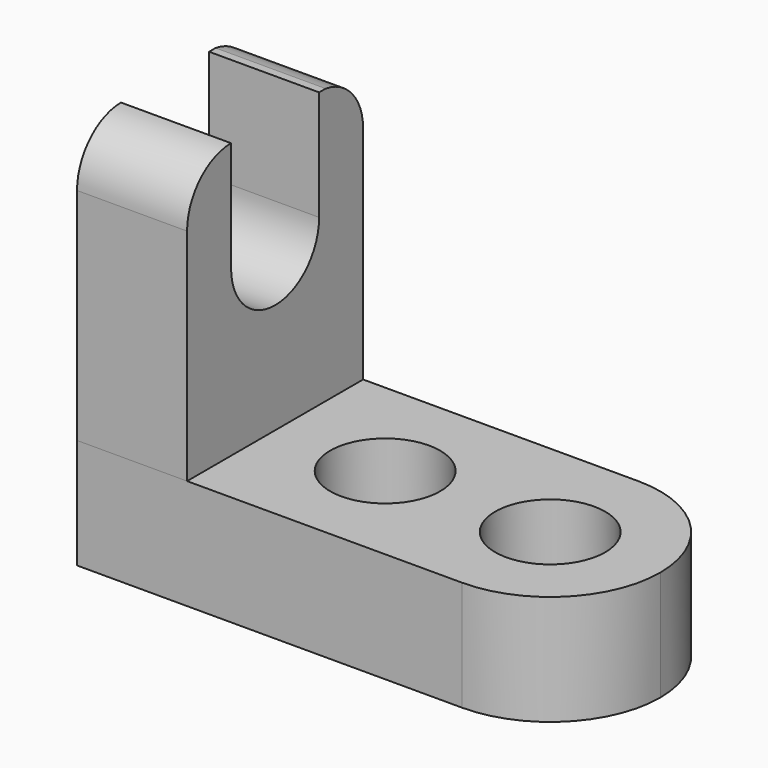
from build123d import *

# Parameters (mm, degrees)
F0_W      = 57.15
F0_H      = 12.7
F1_DEPTH  = 25.4
F2_W      = 12.7
F2_H      = 25.4
F3_DEPTH  = 31.75
F5_DEPTH  = 25.4
F8_DEPTH  = 25.4
F9_DEPTH  = 25.4
F10_R     = 6.35
F11_DEPTH = 25.4
F13_DEPTH = 25.4


with BuildPart() as f1:
    # F0 (on Front) → F1 (new body)
    with BuildSketch(Plane.XZ):
        with Locations((-8.1138868551, 6.35)):
            Rectangle(F0_W, F0_H)
    extrude(amount=F1_DEPTH)

    # F10 (on face) → F11 (cut)
    with BuildSketch(Plane.XY.offset(12.7)):
        with Locations((-11.2888868551, -12.7)):
            Circle(F10_R)
        with Locations((7.7611131449, -12.7)):
            Circle(F10_R)
    extrude(amount=-F11_DEPTH, mode=Mode.SUBTRACT)

    # F12 (on face) → F13 (cut)
    with BuildSketch(Plane.XY.offset(12.7)):
        with BuildLine():
            ThreePointArc((20.4611131449, -12.7), (16.741369266, -21.6802561211), (7.7611131449, -25.4))
            Line((7.7611131449, -25.4), (20.4611131449, -25.4))
            Line((20.4611131449, -25.4), (20.4611131449, -12.7))
        make_face()
        with BuildLine():
            ThreePointArc((7.7611131449, 0), (16.741369266, -3.7197438789), (20.4611131449, -12.7))
            Line((20.4611131449, -12.7), (20.4611131449, 0))
            Line((20.4611131449, 0), (7.7611131449, 0))
        make_face()
    extrude(amount=-F13_DEPTH, mode=Mode.SUBTRACT)


with BuildPart() as f3:
    # F2 (on face) → F3 (new body)
    with BuildSketch(Plane.XY.offset(12.7)):
        with Locations((-30.3388868551, -12.7)):
            Rectangle(F2_W, F2_H)
    extrude(amount=F3_DEPTH)

    # F4 (on face) → F5 (cut)
    with BuildSketch(Plane.YZ.offset(-23.9888868551)):
        with BuildLine():
            ThreePointArc((-19.05, 31.75), (-12.7, 38.1), (-6.35, 31.75))
            Line((-6.35, 31.75), (-6.35, 44.45))
            Line((-6.35, 44.45), (-19.05, 44.45))
            Line((-19.05, 44.45), (-19.05, 31.75))
        make_face()
        with BuildLine():
            Line((-19.05, 31.75), (-6.35, 31.75))
            ThreePointArc((-6.35, 31.75), (-12.7, 38.1), (-19.05, 31.75))
        make_face()
        with BuildLine():
            ThreePointArc((-19.05, 31.75), (-12.7, 25.4), (-6.35, 31.75))
            Line((-6.35, 31.75), (-19.05, 31.75))
        make_face()
    extrude(amount=-F5_DEPTH, mode=Mode.SUBTRACT)

    # F6 (on face) → F8 (cut)
    with BuildSketch(Plane.YZ.offset(-23.9888868551)):
        with BuildLine():
            Line((-25.4, 44.45), (-25.4, 38.1))
            ThreePointArc((-25.4, 38.1), (-23.5401280605, 42.5901280605), (-19.05, 44.45))
            Line((-19.05, 44.45), (-25.4, 44.45))
        make_face()
    extrude(amount=-F8_DEPTH, mode=Mode.SUBTRACT)

    # F7 (on face) → F9 (cut)
    with BuildSketch(Plane.YZ.offset(-23.9888868551)):
        with BuildLine():
            ThreePointArc((-5.4130867227, 44.45), (-1.5400156284, 42.3151653979), (0, 38.1694989443))
            Line((0, 38.1694989443), (0, 44.45))
            Line((0, 44.45), (-5.4130867227, 44.45))
        make_face()
    extrude(amount=-F9_DEPTH, mode=Mode.SUBTRACT)


solid = Compound([f1.part, f3.part])
